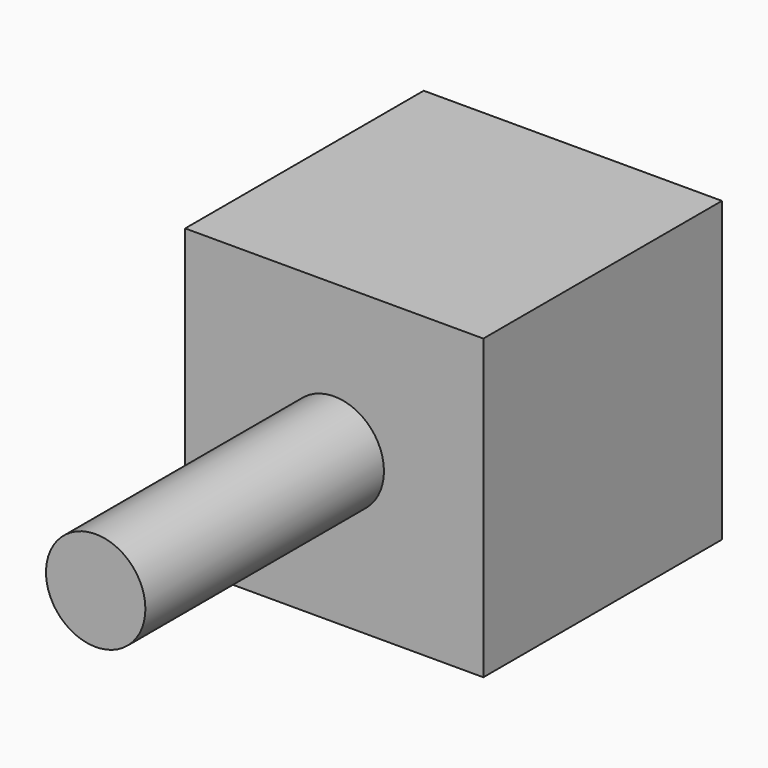
from build123d import *

# Parameters (mm, degrees)
F0_W     = 30
F0_H     = 30
F1_DEPTH = 15
F2_R     = 5
F3_DEPTH = 30


# Not quite as in the source:
# - a feature of the source that left no trace in its solid (it failed there, or was rolled back) is left out


with BuildPart() as f1:
    # F0 (on Top) → F1 (new body, symmetric)
    with BuildSketch(Plane.XY):
        Rectangle(F0_W, F0_H)
    extrude(amount=F1_DEPTH, both=True)

    # F2 (on face) → F3 (join)
    with BuildSketch(Plane.XZ.offset(15)):
        Circle(F2_R)
    extrude(amount=F3_DEPTH)


solid = f1.part
